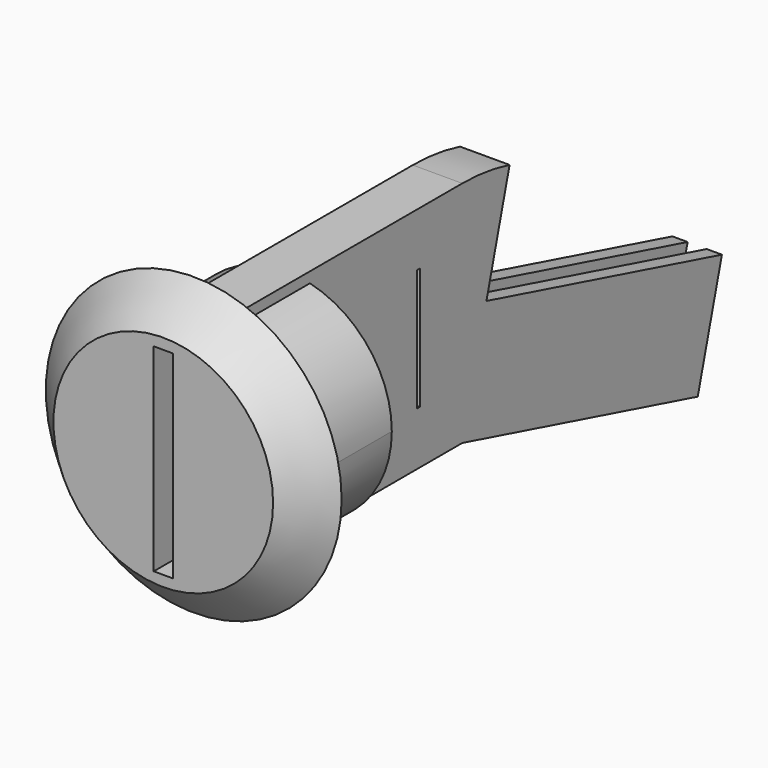
from build123d import *

# Parameters (mm, degrees)
F0_R        = 19.417133546
F0_W        = 2.5
F0_H        = 26
F1_DEPTH    = 5
F2_SIZE     = 4.99999
F3_DEPTH    = 40
F3_FACE_W   = 6.5
F3_FACE_H   = 30
F3_FACE_W_2 = 2.5
F3_FACE_H_2 = 26
F4_ANGLE    = 15
F6_DEPTH    = 40
F7_W        = 0.5
F7_H        = 16
F8_DEPTH    = 25
F9_DEPTH    = 15


# Not quite as in the source:
# - a fillet or chamfer is up to 0.001 mm smaller than in the source, because OpenCascade refuses the exact size


with BuildPart() as f1:
    # F0 (on Front) → F1 (new body)
    with BuildSketch(Plane.XZ):
        Circle(F0_R)
        with BuildLine():
            ThreePointArc((3.25, 13.6175438314), (10.9886304879, 8.6746757864), (14, 0))
            ThreePointArc((14, 0), (10.9886304879, -8.6746757864), (3.25, -13.6175438314))
            Line((3.25, -13.6175438314), (3.25, -15))
            Line((3.25, -15), (-3.25, -15))
            Line((-3.25, -15), (-3.25, -13.6175438314))
            ThreePointArc((-3.25, -13.6175438314), (-14, 0), (-3.25, 13.6175438314))
            Line((-3.25, 13.6175438314), (-3.25, 15))
            Line((-3.25, 15), (3.25, 15))
            Line((3.25, 15), (3.25, 13.6175438314))
        make_face(mode=Mode.SUBTRACT)
        with BuildLine():
            Line((-3.25, -13.6175438314), (-3.25, 13.6175438314))
            ThreePointArc((-3.25, 13.6175438314), (-14, 0), (-3.25, -13.6175438314))
        make_face()
        with BuildLine():
            ThreePointArc((3.25, -13.6175438314), (10.9886304879, -8.6746757864), (14, 0))
            ThreePointArc((14, 0), (10.9886304879, 8.6746757864), (3.25, 13.6175438314))
            Line((3.25, 13.6175438314), (3.25, -13.6175438314))
        make_face()
        with BuildLine():
            Line((3.25, -13.6175438314), (3.25, 13.6175438314))
            ThreePointArc((3.25, 13.6175438314), (0, 14), (-3.25, 13.6175438314))
            Line((-3.25, 13.6175438314), (-3.25, -13.6175438314))
            ThreePointArc((-3.25, -13.6175438314), (0, -14), (3.25, -13.6175438314))
        make_face()
        Rectangle(F0_W, F0_H, mode=Mode.SUBTRACT)
        with BuildLine():
            Line((3.25, -15), (3.25, -13.6175438314))
            ThreePointArc((3.25, -13.6175438314), (0, -14), (-3.25, -13.6175438314))
            Line((-3.25, -13.6175438314), (-3.25, -15))
            Line((-3.25, -15), (3.25, -15))
        make_face()
        with BuildLine():
            ThreePointArc((-3.25, 13.6175438314), (0, 14), (3.25, 13.6175438314))
            Line((3.25, 13.6175438314), (3.25, 15))
            Line((3.25, 15), (-3.25, 15))
            Line((-3.25, 15), (-3.25, 13.6175438314))
        make_face()
    extrude(amount=F1_DEPTH)

    # F2 (size 5 in the source; OpenCascade refuses exactly that, so slightly less here)
    f2_edges = [f1.edges().sort_by_distance(p)[0] for p in [
        (-19.417134, -5, 0),
    ]]
    chamfer(f2_edges, length=F2_SIZE)

    # F0 (on Front) → F3 (join)
    with BuildSketch(Plane.XZ):
        with BuildLine():
            ThreePointArc((-3.25, 13.6175438314), (0, 14), (3.25, 13.6175438314))
            Line((3.25, 13.6175438314), (3.25, 15))
            Line((3.25, 15), (-3.25, 15))
            Line((-3.25, 15), (-3.25, 13.6175438314))
        make_face()
        with BuildLine():
            Line((3.25, -13.6175438314), (3.25, 13.6175438314))
            ThreePointArc((3.25, 13.6175438314), (0, 14), (-3.25, 13.6175438314))
            Line((-3.25, 13.6175438314), (-3.25, -13.6175438314))
            ThreePointArc((-3.25, -13.6175438314), (0, -14), (3.25, -13.6175438314))
        make_face()
        Rectangle(F0_W, F0_H, mode=Mode.SUBTRACT)
        with BuildLine():
            Line((3.25, -15), (3.25, -13.6175438314))
            ThreePointArc((3.25, -13.6175438314), (0, -14), (-3.25, -13.6175438314))
            Line((-3.25, -13.6175438314), (-3.25, -15))
            Line((-3.25, -15), (3.25, -15))
        make_face()
    extrude(amount=-F3_DEPTH)

    # F3_face (on face) → F4 (revolve)
    with BuildSketch(Plane(origin=(0, 40, 0), x_dir=(1, 0, 0), z_dir=(0, 1, 0))):
        Rectangle(F3_FACE_W, F3_FACE_H)
        Rectangle(F3_FACE_W_2, F3_FACE_H_2, mode=Mode.SUBTRACT)
    revolve(axis=Axis((0, 40, -15), (-1, 0, 0)), revolution_arc=F4_ANGLE)

    # F5 (on face) → F6 (join)
    with BuildSketch(Plane(origin=(0, 41.0705080757, -11.0048094716), x_dir=(-1, 0, 0), z_dir=(0, 0.9659258263, -0.2588190451))):
        Polygon((3.25, -4.1361255902), (3.25, 11.1839016899), (1.25, 11.1839016899), (1.25, -2.1361255902), (-1.25, -2.1361255902), (-1.25, 11.1839016899), (-3.25, 11.1839016899), (-3.25, -4.1361255902), align=None)
    extrude(amount=F6_DEPTH)

    # F7 (on face) → F8 (cut)
    with BuildSketch(Plane(origin=(-3.25, 0, 0), x_dir=(0, -1, 0), z_dir=(-1, 0, 0))):
        with Locations((-32.7866710722, 0)):
            Rectangle(F7_W, F7_H)
    extrude(amount=-F8_DEPTH, mode=Mode.SUBTRACT)

    # F0 (on Front) → F9 (join)
    with BuildSketch(Plane.XZ):
        with BuildLine():
            ThreePointArc((3.25, -13.6175438314), (10.9886304879, -8.6746757864), (14, 0))
            ThreePointArc((14, 0), (10.9886304879, 8.6746757864), (3.25, 13.6175438314))
            Line((3.25, 13.6175438314), (3.25, -13.6175438314))
        make_face()
        with BuildLine():
            Line((-3.25, -13.6175438314), (-3.25, 13.6175438314))
            ThreePointArc((-3.25, 13.6175438314), (-14, 0), (-3.25, -13.6175438314))
        make_face()
    extrude(amount=-F9_DEPTH)


solid = f1.part
